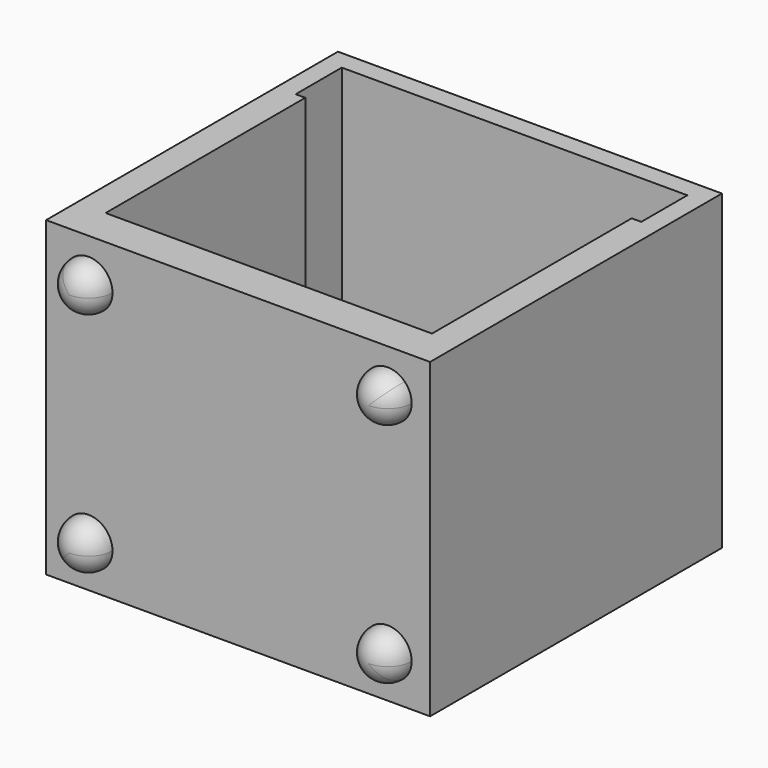
from build123d import *

# Parameters (mm, degrees)
F0_W     = 101.6
F0_H     = 96.52
F1_DEPTH = 82.55
F2_W     = 91.44
F2_H     = 81.28
F3_DEPTH = 77.47
F4_W     = 2.54
F4_H     = 66.04
F5_DEPTH = 81.28
F6_R     = 1.397
F7_DEPTH = 3.302
F9_DEPTH = 6.35
F10_R    = 6.34999


# Not quite as in the source:
# - a fillet or chamfer is up to 0.001 mm smaller than in the source, because OpenCascade refuses the exact size


with BuildPart() as f1:
    # F0 (on Top) → F1 (new body)
    with BuildSketch(Plane.XY):
        Rectangle(F0_W, F0_H)
    extrude(amount=F1_DEPTH)

    # F2 (on face) → F3 (cut)
    with BuildSketch(Plane.XY.offset(82.55)):
        with Locations((0, 2.54)):
            Rectangle(F2_W, F2_H)
    extrude(amount=-F3_DEPTH, mode=Mode.SUBTRACT)

    # F4 (on face) → F5 (join)
    with BuildSketch(Plane.XY.offset(82.55)):
        with Locations((-44.45, -5.08)):
            Rectangle(F4_W, F4_H)
        with Locations((44.45, -5.08)):
            Rectangle(F4_W, F4_H)
    extrude(amount=-F5_DEPTH)

    # F6 (on face) → F7 (cut)
    with BuildSketch(Plane(origin=(0, 48.26, 0), x_dir=(-1, 0, 0), z_dir=(0, 1, 0))):
        with Locations((-46.3098719395, 78.0598719395)):
            Circle(F6_R)
        with Locations((46.3098719395, 78.0598719395)):
            Circle(F6_R)
        with Locations((46.3098719395, 4.4901280605)):
            Circle(F6_R)
        with Locations((-46.3098719395, 4.4901280605)):
            Circle(F6_R)
    extrude(amount=-F7_DEPTH, mode=Mode.SUBTRACT)

    # F8 (on face) → F9 (join)
    with BuildSketch(Plane.XZ.offset(48.26)):
        with BuildLine():
            ThreePointArc((-44.0648079092, 75.8148079092), (-42.0047196442, 65.4580448172), (-33.2246798487, 71.3246798487))
            ThreePointArc((-33.2246798487, 71.3246798487), (-37.1446400531, 77.1913148801), (-44.0648079092, 75.8148079092))
        make_face()
        with BuildLine():
            ThreePointArc((44.0648079092, 75.8148079092), (33.7080448172, 68.8946400531), (45.9246798487, 71.3246798487))
            ThreePointArc((45.9246798487, 71.3246798487), (45.4413148801, 73.7547196442), (44.0648079092, 75.8148079092))
        make_face()
        with BuildLine():
            ThreePointArc((44.0648079092, 6.7351920908), (45.4413148801, 8.7952803558), (45.9246798487, 11.2253201513))
            ThreePointArc((45.9246798487, 11.2253201513), (33.7080448172, 13.6553599469), (44.0648079092, 6.7351920908))
        make_face()
        with BuildLine():
            ThreePointArc((-44.0648079092, 6.7351920908), (-37.1446400531, 5.3586851199), (-33.2246798487, 11.2253201513))
            ThreePointArc((-33.2246798487, 11.2253201513), (-42.0047196442, 17.0919551828), (-44.0648079092, 6.7351920908))
        make_face()
    extrude(amount=F9_DEPTH)

    # F10 (radius 6.35 in the source; OpenCascade refuses exactly that, so slightly less here)
    f10_edges = [f1.edges().sort_by_distance(p)[0] for p in [
        (-45.92468, -54.61, 71.32468),
        (33.22468, -54.61, 71.32468),
        (35.084552, -54.61, 15.715448),
        (-35.084552, -54.61, 15.715448),
    ]]
    fillet(f10_edges, radius=F10_R)


solid = f1.part
